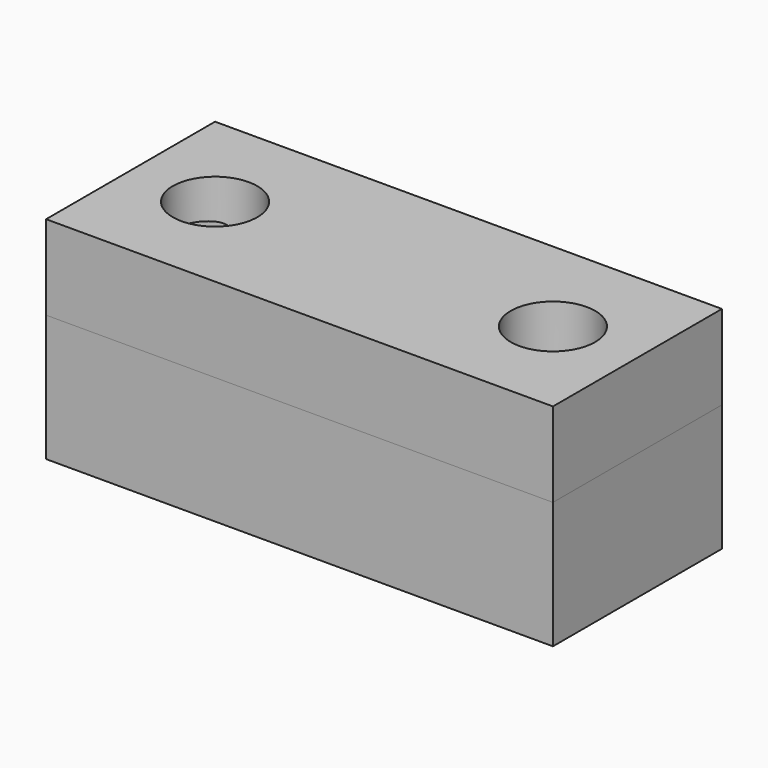
from build123d import *

# Parameters (mm, degrees)
F0_W     = 60
F0_H     = 15
F1_DEPTH = 12.5
F4_W     = 1
F4_H     = 12
F6_W     = 60
F6_H     = 10
F7_DEPTH = 12.5
F8_W     = 5
F8_H     = 10
F12_W    = 1
F12_H    = 12


# Not quite as in the source:
# - a pattern or mirror of a feature is missing from the dataset's text; its kind, count and spacing are read off the source's solid


with BuildPart() as f1:
    # F0 (on Front) → F1 (new body, symmetric)
    with BuildSketch(Plane.XZ):
        with Locations((0, -7.5)):
            Rectangle(F0_W, F0_H)
    extrude(amount=F1_DEPTH, both=True)

    # F2 (on Front) → F3 (revolve, cut)
    with BuildSketch(Plane.XZ):
        Polygon((-21.9591817715, -12.4931969619), (-18.7036573682, -13.778055791), (-22, 6), (-24.9591817715, 5.5068030381), align=None)
    f3 = revolve(axis=Axis((-20.3518286841, 0, -3.8890278955), (-0.1643989873, 0, 0.9863939238)), mode=Mode.SUBTRACT)

    # F3_copies: F3 across plane
    add(f3.mirror(Plane(origin=(0, 0, 0), x_dir=(0, 0, 1), z_dir=(1, 0, 0))), mode=Mode.SUBTRACT)


with BuildPart() as f5:
    # F4 (on Front) → F5 (revolve)
    with BuildSketch(Plane.XZ):
        with Locations((-20.5, -6)):
            Rectangle(F4_W, F4_H)
    revolve(axis=Axis((-20, 0, -6), (0, 0, -1)))


with BuildPart() as f7:
    # F6 (on Front) → F7 (new body, symmetric)
    with BuildSketch(Plane.XZ):
        with Locations((0, 5)):
            Rectangle(F6_W, F6_H)
    extrude(amount=F7_DEPTH, both=True)

    # F8 (on Front) → F9 (revolve, cut)
    with BuildSketch(Plane.XZ):
        with Locations((-22.5, 5)):
            Rectangle(F8_W, F8_H)
    f9 = revolve(axis=Axis((-20, 0, 5), (0, 0, 1)), mode=Mode.SUBTRACT)

    # F9_copies: F9 across plane
    add(f9.mirror(Plane(origin=(0, 0, 0), x_dir=(0, 0, 1), z_dir=(1, 0, 0))), mode=Mode.SUBTRACT)


with BuildPart() as f11:
    # F10 (on Front) → F11 (revolve)
    with BuildSketch(Plane.XZ):
        Polygon((-24.9591817715, 5.5068030381), (-22.3287979746, -10.2754997432), (-19.3696162031, -9.7823027813), (-22, 6), align=None)
    revolve(axis=Axis((-20.6848081016, 0, -1.8911513907), (0.1643989873, 0, -0.9863939238)))


with BuildPart() as f11_copies_1:
    # F11_copies: instance of F11
    add(f11.part.mirror(Plane(origin=(0, 0, 0), x_dir=(0, 0, 1), z_dir=(1, 0, 0))))


with BuildPart() as f11_1:
    add(f11.part)

    # F12 (on Front) → F13 (revolve, cut)
    with BuildSketch(Plane.XZ):
        with Locations((-20.5, -6)):
            Rectangle(F12_W, F12_H)
    revolve(axis=Axis((-20, 0, -6), (0, 0, 1)), mode=Mode.SUBTRACT)


solid = Compound([f1.part, f5.part, f7.part, f11_copies_1.part, f11_1.part])
